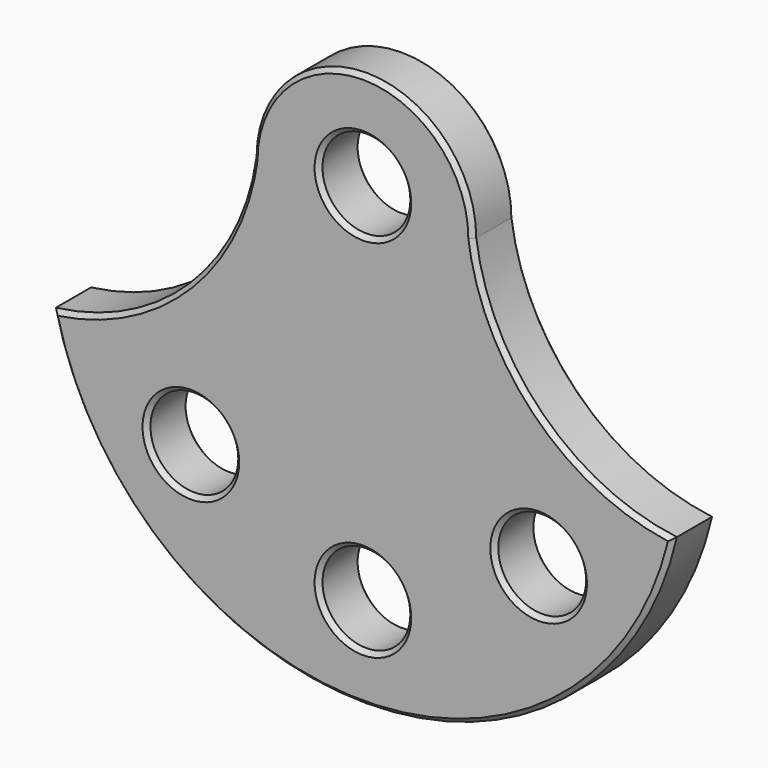
from build123d import *

# Parameters (mm, degrees)
F1_DEPTH   = 12
F3_D       = 20
F4_C1_SIZE = 1
F4_C2_SIZE = 1
F4_C3_SIZE = 1
F4_C4_SIZE = 1
F4_C5_SIZE = 1
F4_C6_SIZE = 1
F4_C7_SIZE = 1
F4_C8_SIZE = 0.9999
F5_C1_SIZE = 1
F5_C2_SIZE = 1
F5_C3_SIZE = 1
F5_C4_SIZE = 1
F5_C5_SIZE = 1
F5_C6_SIZE = 1
F5_C7_SIZE = 1
F5_C8_SIZE = 0.9999


# Not quite as in the source:
# - a fillet or chamfer is up to 0.001 mm smaller than in the source, because OpenCascade refuses the exact size


with BuildPart() as f1:
    # F0 (on Front) → F1 (new body)
    with BuildSketch(Plane.XZ):
        with BuildLine():
            ThreePointArc((-70.6781876117, 0), (0, -56.3108485805), (70.6781876117, 0))
            ThreePointArc((70.6781876117, 0), (40.1621081353, 14.7607018174), (25, 45.079341326))
            ThreePointArc((25, 45.079341326), (0, 20.079341326), (-25, 45.079341326))
            ThreePointArc((-25, 45.079341326), (-40.2089612492, 14.808177341), (-70.6781876117, 0))
        make_face()
        with BuildLine():
            ThreePointArc((-25, 45.079341326), (0, 20.079341326), (25, 45.079341326))
            Line((25, 45.079341326), (-25, 45.079341326))
        make_face()
        with BuildLine():
            Line((-25, 45.079341326), (25, 45.079341326))
            ThreePointArc((25, 45.079341326), (0, 70.079341326), (-25, 45.079341326))
        make_face()
    extrude(amount=F1_DEPTH)

    # F3 (through all)
    with Locations(Plane(origin=(0, 0, 0), x_dir=(-1, 0, 0), z_dir=(0, 1, 0))):
        with Locations((-40.0044433773, -15.3863234445), (0, -35.2486670017), (39.1651876271, -16.7850796133), (0, 47.8374771774)):
            Hole(F3_D / 2)

    # F4: chamfer of 1 on 8 edges, made by hand

    # F4_c1
    f4_c1_edges = [f1.edges().sort_by_distance(p)[0] for p in [
        (40.1621081353, 0, 14.7607018174),
    ]]
    chamfer(f4_c1_edges, length=F4_C1_SIZE)

    # F4_c2
    f4_c2_edges = [f1.edges().sort_by_distance(p)[0] for p in [
        (-0.5029833863, 0, -56.3091040511),
    ]]
    chamfer(f4_c2_edges, length=F4_C2_SIZE)

    # F4_c3
    f4_c3_edges = [f1.edges().sort_by_distance(p)[0] for p in [
        (-39.8532973479, 0, 15.1625303947),
    ]]
    chamfer(f4_c3_edges, length=F4_C3_SIZE)

    # F4_c4
    f4_c4_edges = [f1.edges().sort_by_distance(p)[0] for p in [
        (10, 0, -35.2486670017),
    ]]
    chamfer(f4_c4_edges, length=F4_C4_SIZE)

    # F4_c5
    f4_c5_edges = [f1.edges().sort_by_distance(p)[0] for p in [
        (-29.1651876271, 0, -16.7850796133),
    ]]
    chamfer(f4_c5_edges, length=F4_C5_SIZE)

    # F4_c6
    f4_c6_edges = [f1.edges().sort_by_distance(p)[0] for p in [
        (50.0044433773, 0, -15.3863234445),
    ]]
    chamfer(f4_c6_edges, length=F4_C6_SIZE)

    # F4_c7
    f4_c7_edges = [f1.edges().sort_by_distance(p)[0] for p in [
        (10, 0, 47.8374771774),
    ]]
    chamfer(f4_c7_edges, length=F4_C7_SIZE)

    # F4_c8 (size 1 in the source; OpenCascade refuses exactly that, so slightly less here)
    f4_c8_edges = [f1.edges().sort_by_distance(p)[0] for p in [
        (0, 0, 70.079341326),
    ]]
    chamfer(f4_c8_edges, length=F4_C8_SIZE)

    # F5: chamfer of 1 on 8 edges, made by hand

    # F5_c1
    f5_c1_edges = [f1.edges().sort_by_distance(p)[0] for p in [
        (40.1621081353, -12, 14.7607018174),
    ]]
    chamfer(f5_c1_edges, length=F5_C1_SIZE)

    # F5_c2
    f5_c2_edges = [f1.edges().sort_by_distance(p)[0] for p in [
        (-0.5029833863, -12, -56.3091040511),
    ]]
    chamfer(f5_c2_edges, length=F5_C2_SIZE)

    # F5_c3
    f5_c3_edges = [f1.edges().sort_by_distance(p)[0] for p in [
        (-39.8532973479, -12, 15.1625303947),
    ]]
    chamfer(f5_c3_edges, length=F5_C3_SIZE)

    # F5_c4
    f5_c4_edges = [f1.edges().sort_by_distance(p)[0] for p in [
        (10, -12, 47.8374771774),
    ]]
    chamfer(f5_c4_edges, length=F5_C4_SIZE)

    # F5_c5
    f5_c5_edges = [f1.edges().sort_by_distance(p)[0] for p in [
        (50.0044433773, -12, -15.3863234445),
    ]]
    chamfer(f5_c5_edges, length=F5_C5_SIZE)

    # F5_c6
    f5_c6_edges = [f1.edges().sort_by_distance(p)[0] for p in [
        (-29.1651876271, -12, -16.7850796133),
    ]]
    chamfer(f5_c6_edges, length=F5_C6_SIZE)

    # F5_c7
    f5_c7_edges = [f1.edges().sort_by_distance(p)[0] for p in [
        (10, -12, -35.2486670017),
    ]]
    chamfer(f5_c7_edges, length=F5_C7_SIZE)

    # F5_c8 (size 1 in the source; OpenCascade refuses exactly that, so slightly less here)
    f5_c8_edges = [f1.edges().sort_by_distance(p)[0] for p in [
        (0, -12, 70.079341326),
    ]]
    chamfer(f5_c8_edges, length=F5_C8_SIZE)


solid = f1.part
